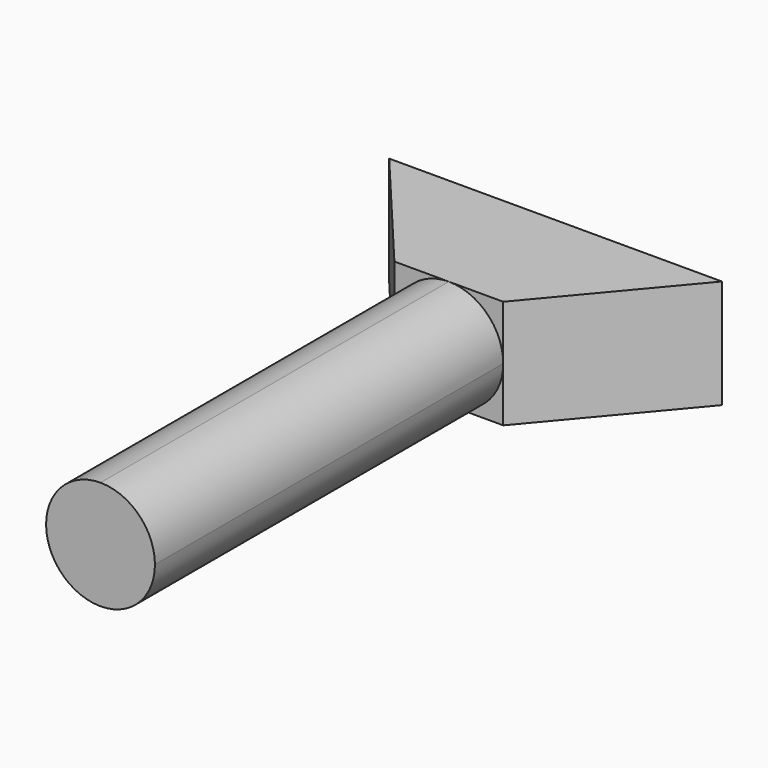
from build123d import *

# Parameters (mm, degrees)
F1_DEPTH = 31.75
F3_DEPTH = 127


# Not quite as in the source:
# - a feature names something its author has since deleted; it is built from what else it names


with BuildPart() as f1:
    # F0 (on Top) → F1 (new body)
    with BuildSketch(Plane.XY):
        Polygon((-48.5286105721, 38.9150577104), (-15.875, 0), (15.875, 0), (48.5286105721, 38.9150577104), align=None)
    extrude(amount=F1_DEPTH)

    # F2 (on face) → F3 (join)
    with BuildSketch(Plane.XZ):
        with BuildLine():
            ThreePointArc((5.44e-08, 0), (11.2253201706, 4.6496798679), (15.875, 15.875))
            ThreePointArc((15.875, 15.875), (11.2253201513, 27.1003201513), (0, 31.75))
            ThreePointArc((0, 31.75), (-11.2253201513, 27.1003201513), (-15.875, 15.875))
            ThreePointArc((-15.875, 15.875), (-11.2253201321, 4.6496798294), (5.44e-08, 0))
        make_face()
    extrude(amount=F3_DEPTH)


solid = f1.part
